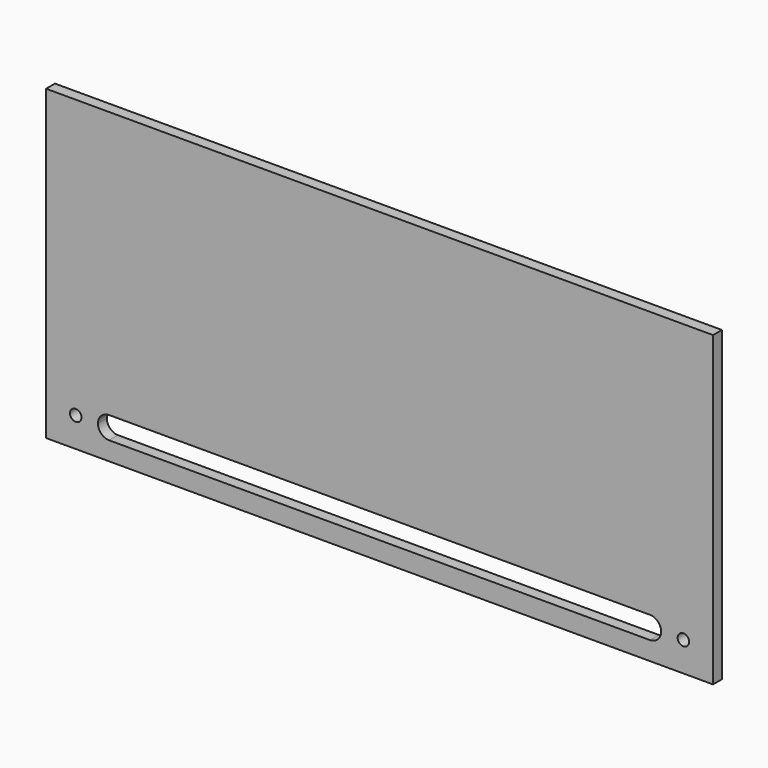
from build123d import *

# Parameters (mm, degrees)
F0_W     = 180
F0_H     = 83
F1_DEPTH = 3
F2_R     = 1.55
F2_W     = 152
F2_H     = 6
F3_DEPTH = 25
F4_R     = 2.99999


# Not quite as in the source:
# - a fillet or chamfer is up to 0.001 mm smaller than in the source, because OpenCascade refuses the exact size


with BuildPart() as f1:
    # F0 (on Front) → F1 (new body)
    with BuildSketch(Plane.XZ):
        with Locations((98.9931351204, 58.851495102)):
            Rectangle(F0_W, F0_H)
    extrude(amount=F1_DEPTH)

    # F2 (on face) → F3 (cut)
    with BuildSketch(Plane.XZ.offset(3)):
        with Locations((180.9931351204, 25.351495102)):
            Circle(F2_R)
        with Locations((98.9931351204, 25.351495102)):
            Rectangle(F2_W, F2_H)
        with Locations((16.9931351204, 25.351495102)):
            Circle(F2_R)
    extrude(amount=-F3_DEPTH, mode=Mode.SUBTRACT)

    # F4 (radius 3 in the source; OpenCascade refuses exactly that, so slightly less here)
    f4_edges = [f1.edges().sort_by_distance(p)[0] for p in [
        (22.993135, -1.5, 28.351495),
        (22.993135, -1.5, 22.351495),
        (174.993135, -1.5, 28.351495),
        (174.993135, -1.5, 22.351495),
    ]]
    fillet(f4_edges, radius=F4_R)


solid = f1.part
